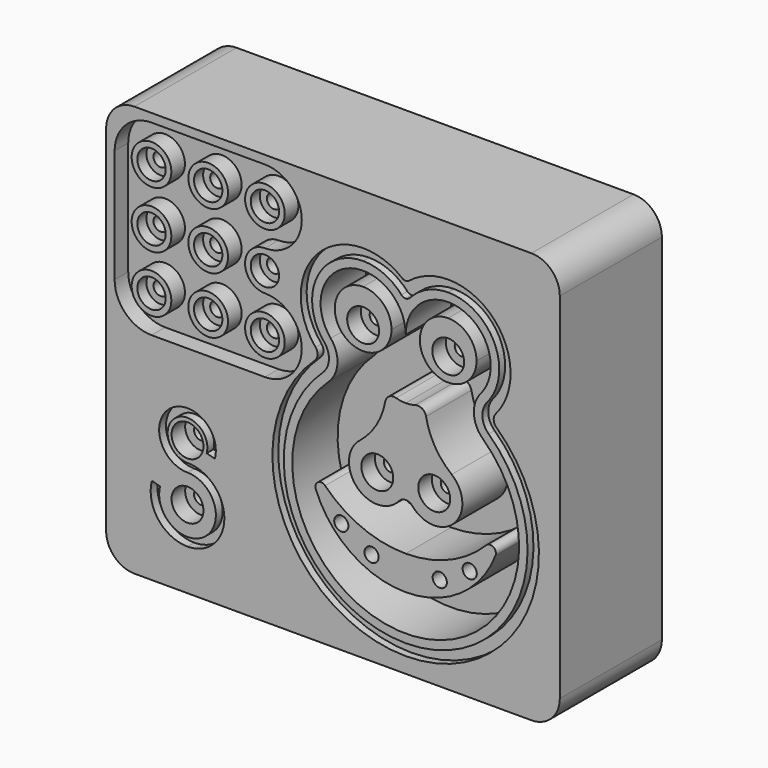
from build123d import *

# Parameters (mm, degrees)
F1_DEPTH              = 45
F4_DEPTH              = 5
F5_R                  = 20
F5_R_2                = 15
F5_R_3                = 12
F5_R_4                = 10
F5_R_5                = 8
F5_R_6                = 14
F5_R_7                = 11
F6_DEPTH              = 10
F9_DEPTH              = 6
F10_R                 = 7
F11_DEPTH             = 6
F13_D                 = 5
F13_DEPTH             = 19.48
F13_CBORE_D           = 10
F13_CBORE_DEPTH       = 4
F13_TIP               = 1.5021515476
F13_ON_F8_D           = 5
F13_ON_F8_DEPTH       = 19.48
F13_ON_F8_CBORE_D     = 10
F13_ON_F8_CBORE_DEPTH = 4
F13_ON_F8_TIP         = 1.5021515476
F15_DEPTH             = 2.6
F17_DEPTH             = 20
F20_DEPTH             = 20
F22_D                 = 5
F22_DEPTH             = 15
F22_CBORE_D           = 11.25
F22_CBORE_DEPTH       = 6
F22_TIP               = 1.5021515476
F26_DEPTH             = 3
F28_D                 = 5
F28_DEPTH             = 18
F28_CBORE_D           = 11.25
F28_CBORE_DEPTH       = 6
F28_TIP               = 1.5021515476
F30_D                 = 5
F30_DEPTH             = 15
F30_CBORE_D           = 11.25
F30_CBORE_DEPTH       = 6
F30_TIP               = 1.5021515476
F31_D                 = 5
F31_DEPTH             = 15
F31_TIP               = 1.5021515476
F31_ON_F23_D          = 5
F31_ON_F23_DEPTH      = 15
F31_ON_F23_TIP        = 1.5021515476


with BuildPart() as f1:
    # F0 (on Front) → F1 (new body)
    with BuildSketch(Plane.XZ):
        with BuildLine():
            ThreePointArc((80, 62.5), (77.0710678119, 69.5710678119), (70, 72.5))
            Line((70, 72.5), (-70, 72.5))
            ThreePointArc((-70, 72.5), (-77.0710678119, 69.5710678119), (-80, 62.5))
            Line((-80, 62.5), (-80, -62.5))
            ThreePointArc((-80, -62.5), (-77.0710678119, -69.5710678119), (-70, -72.5))
            Line((-70, -72.5), (70, -72.5))
            ThreePointArc((70, -72.5), (77.0710678119, -69.5710678119), (80, -62.5))
            Line((80, -62.5), (80, 62.5))
        make_face()
    extrude(amount=-F1_DEPTH)

    # F3 (on face) → F4 (cut)
    with BuildSketch(Plane(origin=(0, 45, 0), x_dir=(-1, 0, 0), z_dir=(0, 1, 0))):
        with BuildLine():
            ThreePointArc((-76, -53.5), (-71.6066017178, -64.1066017178), (-61, -68.5))
            Line((-61, -68.5), (61, -68.5))
            ThreePointArc((61, -68.5), (71.6066017178, -64.1066017178), (76, -53.5))
            Line((76, -53.5), (76, 53.5))
            ThreePointArc((76, 53.5), (71.6066017178, 64.1066017178), (61, 68.5))
            Line((61, 68.5), (-61, 68.5))
            ThreePointArc((-61, 68.5), (-71.6066017178, 64.1066017178), (-76, 53.5))
            Line((-76, 53.5), (-76, -53.5))
        make_face()
    extrude(amount=-F4_DEPTH, mode=Mode.SUBTRACT)

    # F5 (on offset) → F6 (join)
    with BuildSketch(Plane.XZ.offset(-40)):
        with Locations((-40, 30)):
            Circle(F5_R)
        with Locations((-40, 30)):
            Circle(F5_R_2, mode=Mode.SUBTRACT)
        with Locations((40, 30)):
            Circle(F5_R_2)
        with Locations((40, 30)):
            Circle(F5_R_3, mode=Mode.SUBTRACT)
        with Locations((-40, -30)):
            Circle(F5_R_4)
        with Locations((-40, -30)):
            Circle(F5_R_5, mode=Mode.SUBTRACT)
        with Locations((40, -30)):
            Circle(F5_R_6)
        with Locations((40, -30)):
            Circle(F5_R_7, mode=Mode.SUBTRACT)
    extrude(amount=-F6_DEPTH)

    # F8 (on face) → F9 (cut)
    with BuildSketch(Plane.XZ):
        with BuildLine():
            Line((-24, 69.5), (-64, 69.5))
            ThreePointArc((-64, 69.5), (-73.1923881554, 65.6923881554), (-77, 56.5))
            Line((-77, 56.5), (-77, 16.5))
            ThreePointArc((-77, 16.5), (-73.1923881554, 7.3076118446), (-64, 3.5))
            Line((-64, 3.5), (-24, 3.5))
            ThreePointArc((-24, 3.5), (-11, 16.5000060361), (-24.0000120722, 29.5))
            ThreePointArc((-24.0000120722, 29.5), (-31.0000120722, 36.5), (-24.0000120722, 43.5))
            ThreePointArc((-24.0000120722, 43.5), (-11, 56.4999939639), (-24, 69.5))
        make_face()
    extrude(amount=-F9_DEPTH, mode=Mode.SUBTRACT)

    # F10 (on face) → F11 (join)
    with BuildSketch(Plane.XZ):
        with Locations((-44, 56.5)):
            Circle(F10_R)
        with Locations((-44, 36.5)):
            Circle(F10_R)
        with Locations((-44, 16.5)):
            Circle(F10_R)
        with Locations((-64, 56.5)):
            Circle(F10_R)
        with Locations((-64, 36.5)):
            Circle(F10_R)
        with Locations((-64, 16.5)):
            Circle(F10_R)
        with Locations((-24, 56.5)):
            Circle(F10_R)
        with Locations((-24, 16.5)):
            Circle(F10_R)
    extrude(amount=-F11_DEPTH)

    # F13
    with Locations(Plane.XZ):
        with Locations((-64, 56.5), (-44, 56.5), (-24, 56.5), (-64, 36.5), (-44, 16.5), (-24, 16.5), (-64, 16.5)):
            CounterBoreHole(F13_D / 2, F13_CBORE_D / 2, F13_CBORE_DEPTH, depth=F13_DEPTH)
            with Locations((0, 0, -(F13_DEPTH + F13_TIP / 2))):  # 118° drill point
                Cone(0, F13_D / 2, F13_TIP, mode=Mode.SUBTRACT)

    # F13 on F8
    with Locations(Plane.XZ):
        with Locations((-24.0000120722, 36.5), (-44, 36.5)):
            CounterBoreHole(F13_ON_F8_D / 2, F13_ON_F8_CBORE_D / 2, F13_ON_F8_CBORE_DEPTH, depth=F13_ON_F8_DEPTH)
            with Locations((0, 0, -(F13_ON_F8_DEPTH + F13_ON_F8_TIP / 2))):  # 118° drill point
                Cone(0, F13_ON_F8_D / 2, F13_ON_F8_TIP, mode=Mode.SUBTRACT)

    # F14 (on face) → F15 (cut)
    with BuildSketch(Plane.XZ):
        with BuildLine():
            ThreePointArc((26.89, 49.9737444956), (26.3023824427, 49.6478666811), (25.64, 49.5349939952))
            Line((25.64, 49.5349939952), (25.64, 44.0287565553))
            ThreePointArc((25.64, 44.0287565553), (26.4628756555, 44.2058808998), (27.14, 44.7058808998))
            ThreePointArc((27.14, 44.7058808998), (33.2341191002, 49.2058808998), (40.64, 50.8))
            Line((40.64, 50.8), (40.64, 54.8))
            ThreePointArc((40.64, 54.8), (33.3537931303, 53.558400455), (26.89, 49.9737444956))
        make_face()
        with BuildLine():
            Line((25.64, 44.0287565553), (25.64, 49.5349939952))
            ThreePointArc((25.64, 49.5349939952), (24.9776175573, 49.6478666811), (24.39, 49.9737444956))
            ThreePointArc((24.39, 49.9737444956), (17.9262068697, 53.558400455), (10.64, 54.8))
            Line((10.64, 54.8), (10.64, 50.8))
            ThreePointArc((10.64, 50.8), (18.0458808998, 49.2058808998), (24.14, 44.7058808998))
            ThreePointArc((24.14, 44.7058808998), (24.8171243445, 44.2058808998), (25.64, 44.0287565553))
        make_face()
        with BuildLine():
            Line((10.64, 50.8), (10.64, 54.8))
            ThreePointArc((10.64, 54.8), (-9.3273281686, 42.0361142159), (-6.125502141, 18.5550732554))
            ThreePointArc((-6.125502141, 18.5550732554), (-5.416867645, 16.4366930318), (-6.3686045597, 14.4158282501))
            ThreePointArc((-6.3686045597, 14.4158282501), (25.64, -67), (57.6486045597, 14.4158282501))
            ThreePointArc((57.6486045597, 14.4158282501), (56.696867645, 16.4366930318), (57.405502141, 18.5550732554))
            ThreePointArc((57.405502141, 18.5550732554), (60.6073281686, 42.0361142159), (40.64, 54.8))
            Line((40.64, 54.8), (40.64, 50.8))
            ThreePointArc((40.64, 50.8), (56.9769048652, 40.3568207221), (54.3572290245, 21.1450599362))
            ThreePointArc((54.3572290245, 21.1450599362), (52.7037485338, 16.2021727478), (54.9244680015, 11.4868215905))
            ThreePointArc((54.9244680015, 11.4868215905), (25.64, -63), (-3.6444680015, 11.4868215905))
            ThreePointArc((-3.6444680015, 11.4868215905), (-1.4237485338, 16.2021727478), (-3.0772290245, 21.1450599362))
            ThreePointArc((-3.0772290245, 21.1450599362), (-5.6969048652, 40.3568207221), (10.64, 50.8))
        make_face()
    extrude(amount=-F15_DEPTH, mode=Mode.SUBTRACT)

    # F16 (on face) → F17 (cut)
    with BuildSketch(Plane.XZ):
        with BuildLine():
            ThreePointArc((52.0710241871, 23.0875499469), (45.8137141975, 46.8795128255), (25.64, 32.8))
            ThreePointArc((25.64, 32.8), (5.4662858025, 46.8795128255), (-0.7910241871, 23.0875499469))
            ThreePointArc((-0.7910241871, 23.0875499469), (1.5710907996, 16.0262825348), (-1.6013655827, 9.2900665958))
            ThreePointArc((-1.6013655827, 9.2900665958), (25.64, -60), (52.8813655827, 9.2900665958))
            ThreePointArc((52.8813655827, 9.2900665958), (49.7089092004, 16.0262825348), (52.0710241871, 23.0875499469))
        make_face()
    extrude(amount=-F17_DEPTH, mode=Mode.SUBTRACT)

    # F19 (on offset) → F20 (join)
    with BuildSketch(Plane.XZ.offset(-20)):
        with BuildLine():
            ThreePointArc((10.64, 42.8), (3.5689321881, 25.7289321881), (20.64, 32.8))
            ThreePointArc((20.64, 32.8), (17.7110678119, 39.8710678119), (10.64, 42.8))
        make_face()
        with BuildLine():
            ThreePointArc((40.64, 42.8), (33.5689321881, 25.7289321881), (50.64, 32.8))
            ThreePointArc((50.64, 32.8), (47.7110678119, 39.8710678119), (40.64, 42.8))
        make_face()
        with BuildLine():
            ThreePointArc((25.64, -18.4906138709), (26.9277031257, -18.7764035565), (27.9736065468, -19.5801081778))
            ThreePointArc((27.9736065468, -19.5801081778), (42.8006494723, -20.1396651257), (41.8632142547, -5.3317104693))
            ThreePointArc((41.8632142547, -5.3317104693), (35.9846882244, 1.3736717294), (32.8335520114, 9.7157074093))
            ThreePointArc((32.8335520114, 9.7157074093), (31.4538344241, 11.7290010287), (29.0344226126, 12.0505881944))
            ThreePointArc((29.0344226126, 12.0505881944), (27.3548103939, 11.6836483327), (25.64, 11.5604924133))
            ThreePointArc((25.64, 11.5604924133), (23.9251896061, 11.6836483327), (22.2455773874, 12.0505881944))
            ThreePointArc((22.2455773874, 12.0505881944), (19.8261655759, 11.7290010287), (18.4464479886, 9.7157074093))
            ThreePointArc((18.4464479886, 9.7157074093), (15.2953117756, 1.3736717294), (9.4167857453, -5.3317104693))
            ThreePointArc((9.4167857453, -5.3317104693), (8.4793505277, -20.1396651257), (23.3063934532, -19.5801081778))
            ThreePointArc((23.3063934532, -19.5801081778), (24.3522968743, -18.7764035565), (25.64, -18.4906138709))
        make_face()
        with BuildLine():
            ThreePointArc((25.64, -35.1809402555), (10.2525960135, -32.1028551376), (-2.7666210122, -23.3423301834))
            ThreePointArc((-2.7666210122, -23.3423301834), (-5.2760584564, -23.0729470684), (-6.0511365667, -25.4748416273))
            ThreePointArc((-6.0511365667, -25.4748416273), (6.440096949, -41.2193307082), (25.64, -47.1593285195))
            ThreePointArc((25.64, -47.1593285195), (44.839903051, -41.2193307082), (57.3311365667, -25.4748416273))
            ThreePointArc((57.3311365667, -25.4748416273), (56.5560584564, -23.0729470684), (54.0466210122, -23.3423301834))
            ThreePointArc((54.0466210122, -23.3423301834), (41.0274039865, -32.1028551376), (25.64, -35.1809402555))
        make_face()
    extrude(amount=F20_DEPTH)

    # F22
    with Locations(Plane.XZ):
        with Locations((10.64, 30.8990292251), (40.64, 30.9302173555)):
            CounterBoreHole(F22_D / 2, F22_CBORE_D / 2, F22_CBORE_DEPTH, depth=F22_DEPTH)
            with Locations((0, 0, -(F22_DEPTH + F22_TIP / 2))):  # 118° drill point
                Cone(0, F22_D / 2, F22_TIP, mode=Mode.SUBTRACT)

    # F25 (on face) → F26 (cut)
    with BuildSketch(Plane.XZ):
        with BuildLine():
            Line((-44.538519216, -26.8317333157), (-41.6407417371, -27.608190451))
            ThreePointArc((-41.6407417371, -27.608190451), (-57.3876142901, -17.0864665971), (-51.3, -35.02))
            ThreePointArc((-51.3, -35.02), (-45.1909358491, -52.9370281798), (-60.973126607, -42.48413296))
            Line((-60.973126607, -42.48413296), (-63.8570357418, -41.6553524137))
            ThreePointArc((-63.8570357418, -41.6553524137), (-61.6135934238, -52.9338985771), (-51.3, -58.02))
            ThreePointArc((-51.3, -58.02), (-38.3, -45.02), (-51.3, -32.02))
            ThreePointArc((-51.3, -32.02), (-56.2497474683, -29.9697474683), (-58.3, -25.02))
            ThreePointArc((-58.3, -25.02), (-50.3863166545, -18.0798859704), (-44.538519216, -26.8317333157))
        make_face()
    extrude(amount=-F26_DEPTH, mode=Mode.SUBTRACT)

    # F28
    with Locations(Plane.XZ):
        with Locations((-51.3, -25.02), (-51.3, -45.02)):
            CounterBoreHole(F28_D / 2, F28_CBORE_D / 2, F28_CBORE_DEPTH, depth=F28_DEPTH)
            with Locations((0, 0, -(F28_DEPTH + F28_TIP / 2))):  # 118° drill point
                Cone(0, F28_D / 2, F28_TIP, mode=Mode.SUBTRACT)

    # F30
    with Locations(Plane.XZ):
        with Locations((35.7100255787, -13.156324625), (15.6370233744, -13.1576275453)):
            CounterBoreHole(F30_D / 2, F30_CBORE_D / 2, F30_CBORE_DEPTH, depth=F30_DEPTH)
            with Locations((0, 0, -(F30_DEPTH + F30_TIP / 2))):  # 118° drill point
                Cone(0, F30_D / 2, F30_TIP, mode=Mode.SUBTRACT)

    # F31
    with Locations(Plane.XZ):
        with Locations((2.9387214525, -33.1954993308)):
            Hole(F31_D / 2, depth=F31_DEPTH)
            with Locations((0, 0, -(F31_DEPTH + F31_TIP / 2))):  # 118° drill point
                Cone(0, F31_D / 2, F31_TIP, mode=Mode.SUBTRACT)

    # F31 on F23
    with Locations(Plane.XZ):
        with Locations((13.6102288961, -39.4046604633), (37.6697711039, -39.4046604633), (48.217490534, -33.2812815905)):
            Hole(F31_ON_F23_D / 2, depth=F31_ON_F23_DEPTH)
            with Locations((0, 0, -(F31_ON_F23_DEPTH + F31_ON_F23_TIP / 2))):  # 118° drill point
                Cone(0, F31_ON_F23_D / 2, F31_ON_F23_TIP, mode=Mode.SUBTRACT)


solid = f1.part
